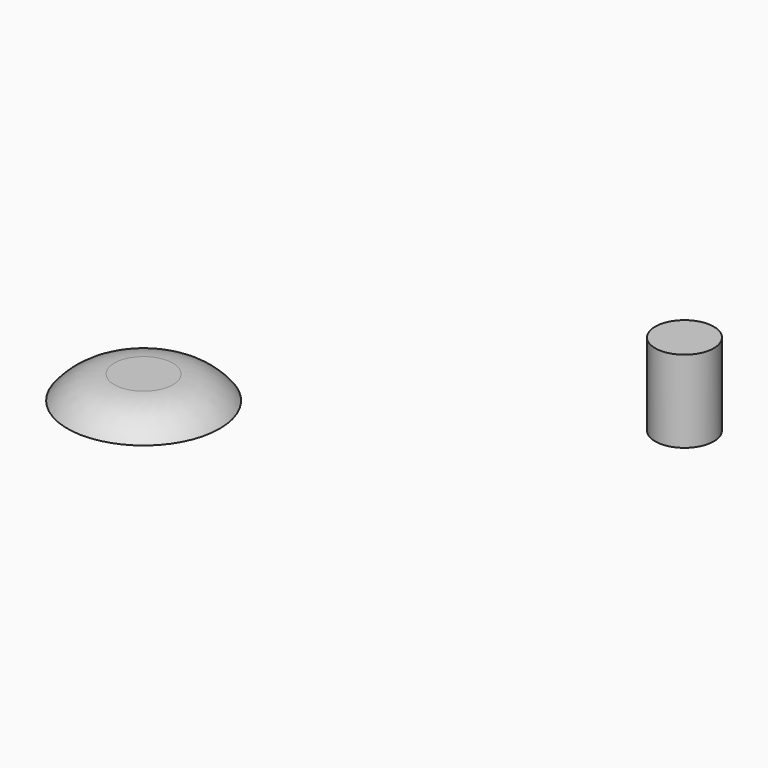
from build123d import *

# Parameters (mm, degrees)
F0_R     = 6.5
F1_DEPTH = 2
F3_R     = 2.5
F4_DEPTH = 7


# Not quite as in the source:
# - a fillet or chamfer that OpenCascade refuses, or shapes differently, is made with other operations: its cross-section is extruded or revolved along the edge and cut away or added


with BuildPart() as f1:
    # F0 (on Top) → F1 (new body)
    with BuildSketch(Plane.XY):
        Circle(F0_R)
    extrude(amount=F1_DEPTH)

    # F2: fillet of radius 5 on 1 edges, made by hand

    # F2_s1 → F2_t2 (revolve, cut)
    with BuildSketch(Plane.XZ):
        with BuildLine():
            ThreePointArc((6.5, 0), (4.7360679775, 1.472135955), (2.5, 2))
            Line((2.5, 2), (6.5, 2))
            Line((6.5, 2), (6.5, 0))
        make_face()
    revolve(axis=Axis((0, 0, 2), (0, 0, 1)), mode=Mode.SUBTRACT)


with BuildPart() as f4:
    # F3 (on Top) → F4 (new body)
    with BuildSketch(Plane.XY):
        with Locations((30.8595001698, 19.1328823566)):
            Circle(F3_R)
    extrude(amount=F4_DEPTH)


solid = Compound([f1.part, f4.part])
